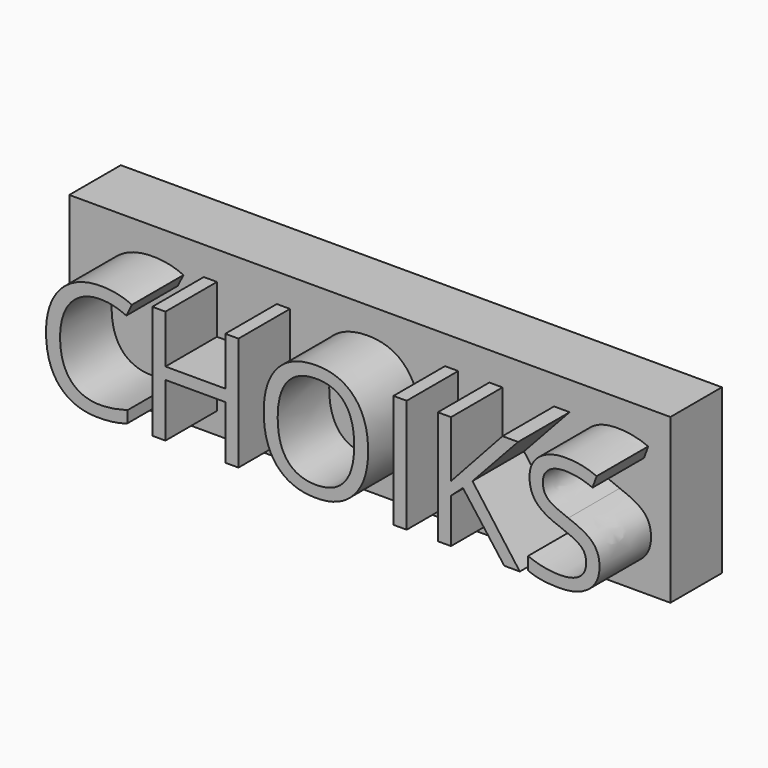
from build123d import *

# Parameters (mm, degrees)
F0_TEXT_SIZE = 61.7439509369
F1_DEPTH     = 25
F2_W         = 233.3467826247
F2_H         = 63.5080672801
F3_DEPTH     = 25


# Not quite as in the source:
# - Text() gives the source's letters only with a copy of the font that has no kerning and outlines rounded to 1/6400 em; it was checked with that copy


with BuildPart() as f1:
    # F0 (on Front) → F1 (new body)
    with BuildSketch(Plane.XZ):
        with Locations((-85.3729955852, -29.3044345453)):
            Text('CHOIKS', F0_TEXT_SIZE, font='Open Sans', text_align=(TextAlign.LEFT, TextAlign.BOTTOM))
    extrude(amount=F1_DEPTH)


with BuildPart() as f3:
    # F2 (on face) → F3 (new body)
    with BuildSketch(Plane(origin=(0, 0, 0), x_dir=(-1, 0, 0), z_dir=(0, 1, 0))):
        with Locations((-24.1050310433, -5.8971773833)):
            Rectangle(F2_W, F2_H)
    extrude(amount=F3_DEPTH)


solid = Compound([f1.part, f3.part])
